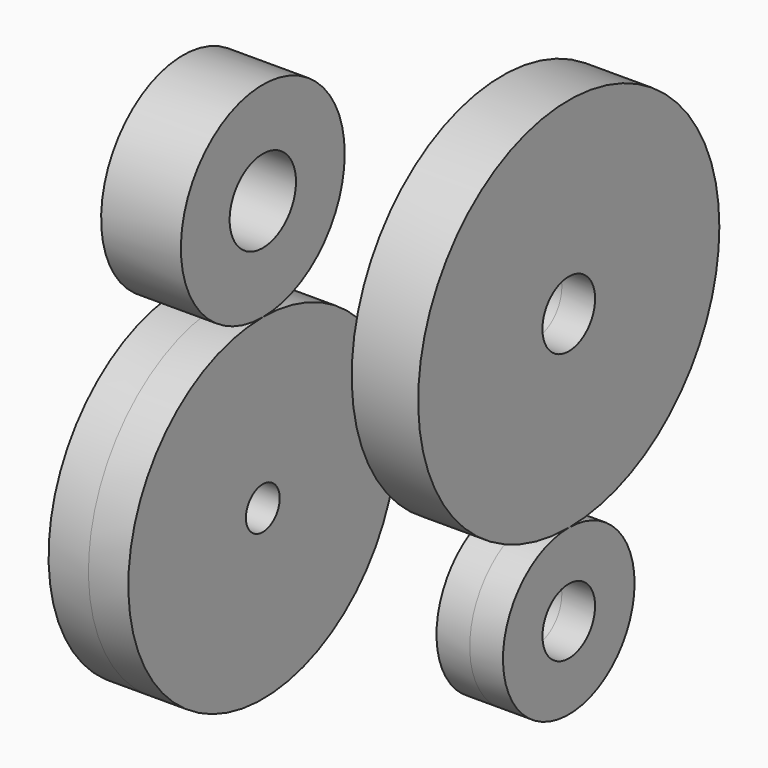
from build123d import *

# Parameters (mm, degrees)
F2_R          = 7.9409001723
F5_DEPTH      = 15
F2_R_2        = 15.5967497012
F6_DEPTH      = 15
F6_DEPTH_BACK = 15
F4_R          = 12.3606629879
F7_DEPTH      = 12.5
F4_R_2        = 12.3779516433
F8_DEPTH      = 12.5


with BuildPart() as f5:
    # F2 (on plane+point) → F5 (new body, symmetric)
    with BuildSketch(Plane.YZ.offset(-58.7768666446)):
        with BuildLine():
            ThreePointArc((63.2045566431, -50.8497282863), (44.6923705955, -6.1573576734), (-2.45e-08, 12.3548283568))
            ThreePointArc((-2.45e-08, 12.3548283568), (-44.6923705955, -95.5420988992), (63.2045566431, -50.8497282863))
        make_face()
        with Locations((0, -50.8497282863)):
            Circle(F2_R, mode=Mode.SUBTRACT)
    extrude(amount=F5_DEPTH, both=True)


with BuildPart() as f6:
    # F2 (on plane+point) → F6 (new body, two sides)
    with BuildSketch(Plane.YZ.offset(-58.7768666446)) as f6_sk:
        with BuildLine():
            ThreePointArc((-2.45e-08, 12.3548283568), (27.2200047725, 23.6297234964), (38.4948999294, 50.8497282863))
            ThreePointArc((38.4948999294, 50.8497282863), (-27.2200047725, 78.0697330761), (-2.45e-08, 12.3548283568))
        make_face()
        with Locations((0, 50.8497282863)):
            Circle(F2_R_2, mode=Mode.SUBTRACT)
    extrude(amount=-F6_DEPTH)
    extrude(f6_sk.sketch, amount=F6_DEPTH_BACK)


with BuildPart() as f7:
    # F4 (on plane+point) → F7 (new body, symmetric)
    with BuildSketch(Plane.YZ.offset(58.7768666446)):
        with BuildLine():
            ThreePointArc((30.9220062538, -50.8497282863), (21.8651603136, -28.98456798), (1.04e-08, -19.9277220325))
            ThreePointArc((1.04e-08, -19.9277220325), (-21.8651603136, -72.7148885925), (30.9220062538, -50.8497282863))
        make_face()
        with Locations((0, -50.8497282863)):
            Circle(F4_R, mode=Mode.SUBTRACT)
    extrude(amount=F7_DEPTH, both=True)

    # F4 (on plane+point) → F8 (join, symmetric)
    with BuildSketch(Plane.YZ.offset(58.7768666446)):
        with BuildLine():
            ThreePointArc((1.04e-08, -19.9277220325), (50.0472150791, 0.8025132145), (70.7774503187, 50.8497282863))
            ThreePointArc((70.7774503187, 50.8497282863), (-50.0472150791, 100.896943358), (1.04e-08, -19.9277220325))
        make_face()
        with Locations((0, 50.8497282863)):
            Circle(F4_R_2, mode=Mode.SUBTRACT)
    extrude(amount=F8_DEPTH, both=True)


solid = Compound([f5.part, f6.part, f7.part])
